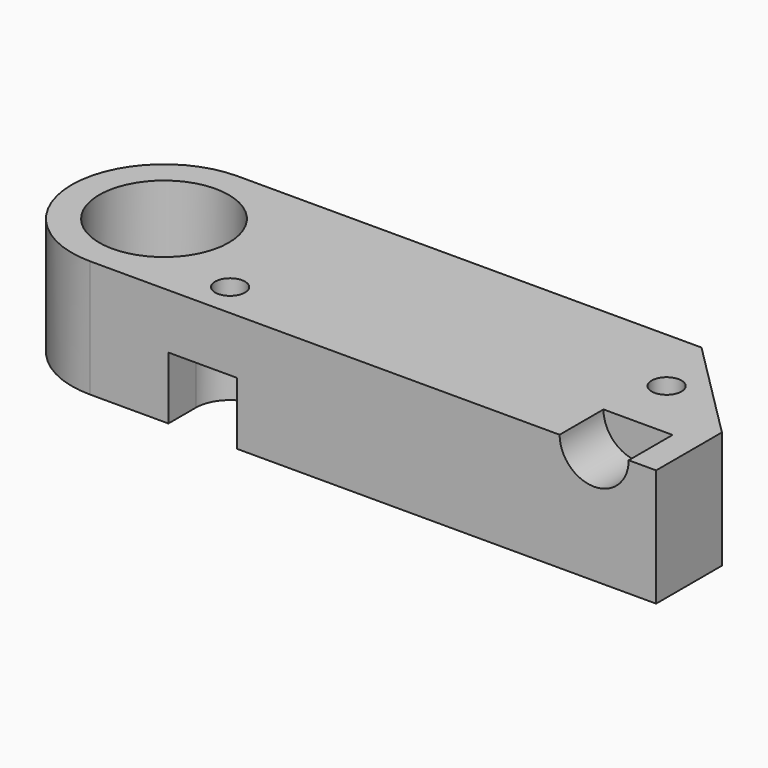
from build123d import *

# Parameters (mm, degrees)
F0_R     = 1.7272
F0_R_2   = 5.9124977
F1_DEPTH = 1.5875
F2_R     = 1.7272
F2_R_2   = 7.5
F3_DEPTH = 12
F5_DEPTH = 6.35
F6_R     = 10.674988
F7_W     = 7.9375
F7_H     = 7.9375
F8_DEPTH = 7.2375014
F9_R     = 3.96874


# Not quite as in the source:
# - a fillet or chamfer is up to 0.001 mm smaller than in the source, because OpenCascade refuses the exact size


with BuildPart() as f1:
    # F0 (on Top) → F1 (new body)
    with BuildSketch(Plane.XY):
        Polygon((64.3750046, 0), (0, 0), (0, -21.3499954), (76.2, -21.3499954), (76.2, -11.8249954), align=None)
        with Locations((23.692892633, -17.3812454)):
            Circle(F0_R, mode=Mode.SUBTRACT)
        with Locations((10.6749977, -10.6749977)):
            Circle(F0_R_2, mode=Mode.SUBTRACT)
        with Locations((66.6185899243, -7.8562454)):
            Circle(F0_R, mode=Mode.SUBTRACT)
    extrude(amount=F1_DEPTH)

    # F2 (on face) → F3 (join)
    with BuildSketch(Plane.XY.offset(1.5875)):
        Polygon((76.2, -21.3499954), (76.2, -11.8249954), (64.3750046, 0), (0, 0), (0, -21.3499954), align=None)
        with Locations((23.692892633, -17.3812454)):
            Circle(F2_R, mode=Mode.SUBTRACT)
        with Locations((10.6749977, -10.6749977)):
            Circle(F2_R_2, mode=Mode.SUBTRACT)
        with Locations((66.6185899243, -7.8562454)):
            Circle(F2_R, mode=Mode.SUBTRACT)
    extrude(amount=F3_DEPTH)

    # F4 (on face) → F5 (cut)
    with BuildSketch(Plane.XZ.offset(21.3499954)):
        with BuildLine():
            Line((73.025, 13.5875), (65.025, 13.5875))
            ThreePointArc((65.025, 13.5875), (69.025, 9.5875), (73.025, 13.5875))
        make_face()
    extrude(amount=-F5_DEPTH, mode=Mode.SUBTRACT)

    # F6 (radius 10.6749977 in the source; OpenCascade refuses exactly that, so slightly less here)
    f6_edges = [f1.edges().sort_by_distance(p)[0] for p in [
        (0, -21.349995, 6.79375),
        (0, 0, 6.79375),
    ]]
    fillet(f6_edges, radius=F6_R)

    # F7 (on face) → F8 (cut)
    with BuildSketch(Plane(origin=(0, 0, 0), x_dir=(1, 0, 0), z_dir=(0, 0, -1))):
        with Locations((23.692892633, 17.3812454)):
            Rectangle(F7_W, F7_H)
        Polygon((62.6498399243, 11.8249954), (62.6498399243, 0), (64.3750046, 0), (70.5873399243, 6.2123353243), (70.5873399243, 11.8249954), align=None)
    extrude(amount=-F8_DEPTH, mode=Mode.SUBTRACT)

    # F9 (radius 3.96875 in the source; OpenCascade refuses exactly that, so slightly less here)
    f9_edges = [f1.edges().sort_by_distance(p)[0] for p in [
        (62.64984, -11.824995, 3.618751),
        (70.58734, -11.824995, 3.618751),
        (19.724143, -13.412495, 3.618751),
        (27.661643, -13.412495, 3.618751),
    ]]
    fillet(f9_edges, radius=F9_R)


solid = f1.part
